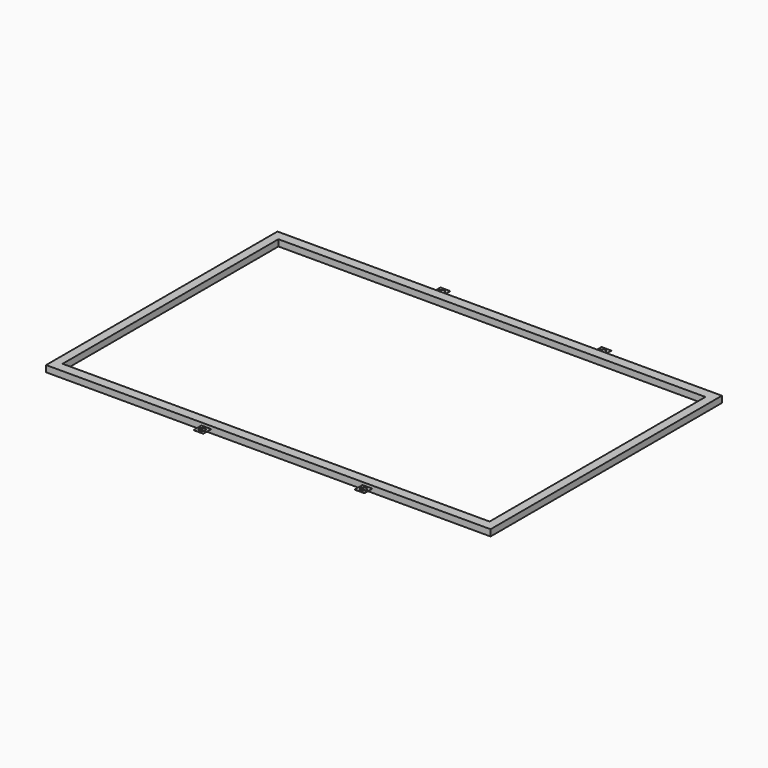
from build123d import *

# Parameters (mm, degrees)
F0_W     = 229
F0_H     = 149
F0_W_2   = 220
F0_H_2   = 139
F1_DEPTH = 3.3
F3_W     = 5
F3_H     = 5
F3_R     = 1.5
F4_DEPTH = 0.1


# Not quite as in the source:
# - a feature names something its author has since deleted; it is built from what else it names


with BuildPart() as f1:
    # F0 (on Top) → F1 (new body)
    with BuildSketch(Plane.XY):
        with Locations((114.5, -74.5)):
            Rectangle(F0_W, F0_H)
        with Locations((114.5, -74.5)):
            Rectangle(F0_W_2, F0_H_2, mode=Mode.SUBTRACT)
    extrude(amount=F1_DEPTH)

    # F3 (on offset) → F4 (join)
    with BuildSketch(Plane.XY.offset(1.8)):
        with Locations((165.5, 2.5)):
            Rectangle(F3_W, F3_H)
        with Locations((165.5, 2.5)):
            Circle(F3_R, mode=Mode.SUBTRACT)
        with Locations((82.5, -151.5)):
            Rectangle(F3_W, F3_H)
        with Locations((82.5, -151.5)):
            Circle(F3_R, mode=Mode.SUBTRACT)
        with Locations((165.5, -151.5)):
            Rectangle(F3_W, F3_H)
        with Locations((165.5, -151.5)):
            Circle(F3_R, mode=Mode.SUBTRACT)
        with Locations((82.5, 2.5)):
            Rectangle(F3_W, F3_H)
        with Locations((82.5, 2.5)):
            Circle(F3_R, mode=Mode.SUBTRACT)
    extrude(amount=F4_DEPTH)


solid = f1.part
